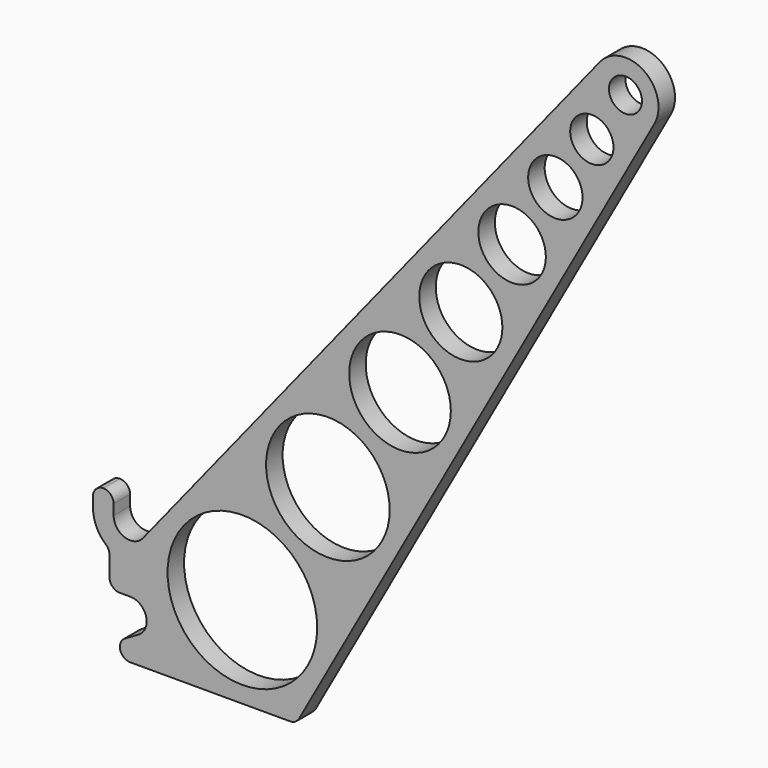
from build123d import *

# Parameters (mm, degrees)
F0_R     = 18.1237353156
F0_R_2   = 14.9714122035
F0_R_3   = 12.3128911041
F0_R_4   = 10.0708194052
F0_R_5   = 8.1799615502
F0_R_6   = 6.5853009382
F0_R_7   = 5.2404391544
F0_R_8   = 4
F1_DEPTH = 5
F2_R     = 2.49999


# Not quite as in the source:
# - a fillet or chamfer is up to 0.001 mm smaller than in the source, because OpenCascade refuses the exact size


with BuildPart() as f1:
    # F0 (on Front) → F1 (new body)
    with BuildSketch(Plane.XZ):
        with BuildLine():
            ThreePointArc((3.1164704126, -2.5075111501), (-1.3293077803, -3.7726569981), (-4, 0))
            Line((-4, 0), (-4, 5))
            Line((-4, 5), (-9, 5))
            Line((-9, 5), (-9, 0))
            ThreePointArc((-9, 0), (-7.9372539332, -4.2426406871), (-5, -7.4833147735))
            Line((-5, -7.4833147735), (-5, -16))
            Line((-5, -16), (0, -16))
            ThreePointArc((0, -16), (2.8284271247, -17.1715728753), (4, -20))
            ThreePointArc((4, -20), (3.4641016151, -22), (2, -23.4641016151))
            Line((2, -23.4641016151), (-9.3205080757, -30))
            Line((-9.3205080757, -30), (40.2062176005, -30))
            Line((40.2062176005, -30), (126.9921824081, 126.1129207402))
            ThreePointArc((126.9921824081, 126.1129207402), (124.4672099784, 136.6365680143), (113.7670591749, 135.0150223001))
            Line((113.7670591749, 135.0150223001), (3.1164704126, -2.5075111501))
        make_face()
        with Locations((27.1926598128, -7.8762646844)):
            Circle(F0_R, mode=Mode.SUBTRACT)
        with Locations((47.9066364562, 22.8967940046)):
            Circle(F0_R_2, mode=Mode.SUBTRACT)
        with Locations((65.375830444, 48.8493448398)):
            Circle(F0_R_3, mode=Mode.SUBTRACT)
        with Locations((80.1085273008, 70.736505998)):
            Circle(F0_R_4, mode=Mode.SUBTRACT)
        with Locations((92.5333911397, 89.1951086458)):
            Circle(F0_R_5, mode=Mode.SUBTRACT)
        with Locations((103.0119371191, 104.7622262472)):
            Circle(F0_R_6, mode=Mode.SUBTRACT)
        with Locations((111.8490501262, 117.8908013099)):
            Circle(F0_R_7, mode=Mode.SUBTRACT)
        with Locations((120, 130)):
            Circle(F0_R_8, mode=Mode.SUBTRACT)
    extrude(amount=F1_DEPTH)

    # F2 (radius 2.5 in the source; OpenCascade refuses exactly that, so slightly less here)
    f2_edges = [f1.edges().sort_by_distance(p)[0] for p in [
        (-9, -2.5, 5),
        (-4, -2.5, 5),
        (-9.320508, -2.5, -30),
        (40.206218, -2.5, -30),
        (-5, -2.5, -7.483315),
        (-5, -2.5, -16),
    ]]
    fillet(f2_edges, radius=F2_R)


solid = f1.part
